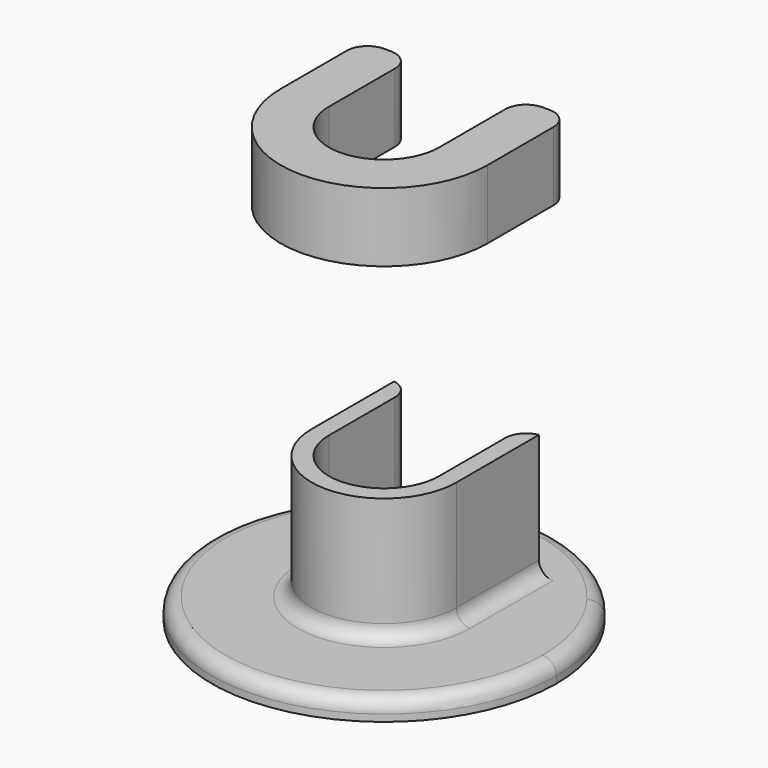
from build123d import *

# Parameters (mm, degrees)
F1_DEPTH = 3
F2_DEPTH = 18
F3_R     = 2
F4_R     = 3
F7_DEPTH = 10
F8_R     = 3


with BuildPart() as f1:
    # F0 (on Top) → F1 (new body)
    with BuildSketch(Plane.XY):
        with BuildLine():
            ThreePointArc((-20, 15), (-7.9056941504, -23.7170824513), (25, 0))
            ThreePointArc((25, 0), (23.7170824513, 7.9056941504), (20, 15))
            Line((20, 15), (10.5, 15))
            Line((10.5, 15), (10.5, 0))
            ThreePointArc((10.5, 0), (0, -10.5), (-10.5, 0))
            Line((-10.5, 0), (-10.5, 15))
            Line((-10.5, 15), (-20, 15))
        make_face()
        with BuildLine():
            Line((10.5, 15), (20, 15))
            ThreePointArc((20, 15), (0, 25), (-20, 15))
            Line((-20, 15), (-10.5, 15))
            Line((-10.5, 15), (-8, 15))
            Line((-8, 15), (8, 15))
            Line((8, 15), (10.5, 15))
        make_face()
        with BuildLine():
            ThreePointArc((-8, 0), (0, -8), (8, 0))
            ThreePointArc((8, 0), (0, 8), (-8, 0))
        make_face()
        with BuildLine():
            Line((8, 0), (8, 6.8007352544))
            ThreePointArc((8, 6.8007352544), (0, 10.5), (-8, 6.8007352544))
            Line((-8, 6.8007352544), (-8, 0))
            ThreePointArc((-8, 0), (0, 8), (8, 0))
        make_face()
        with BuildLine():
            ThreePointArc((-10.5, 0), (0, -10.5), (10.5, 0))
            ThreePointArc((10.5, 0), (9.8552016722, 3.6228441865), (8, 6.8007352544))
            Line((8, 6.8007352544), (8, 0))
            ThreePointArc((8, 0), (0, -8), (-8, 0))
            Line((-8, 0), (-8, 6.8007352544))
            ThreePointArc((-8, 6.8007352544), (-9.8552016722, 3.6228441865), (-10.5, 0))
        make_face()
        with BuildLine():
            Line((-8, 15), (-10.5, 15))
            Line((-10.5, 15), (-10.5, 0))
            ThreePointArc((-10.5, 0), (-9.8552016722, 3.6228441865), (-8, 6.8007352544))
            Line((-8, 6.8007352544), (-8, 15))
        make_face()
        with BuildLine():
            Line((8, 6.8007352544), (8, 15))
            Line((8, 15), (-8, 15))
            Line((-8, 15), (-8, 6.8007352544))
            ThreePointArc((-8, 6.8007352544), (0, 10.5), (8, 6.8007352544))
        make_face()
        with BuildLine():
            Line((10.5, 0), (10.5, 15))
            Line((10.5, 15), (8, 15))
            Line((8, 15), (8, 6.8007352544))
            ThreePointArc((8, 6.8007352544), (9.8552016722, 3.6228441865), (10.5, 0))
        make_face()
    extrude(amount=-F1_DEPTH)

    # F0 (on Top) → F2 (join)
    with BuildSketch(Plane.XY):
        with BuildLine():
            Line((10.5, 0), (10.5, 15))
            Line((10.5, 15), (8, 15))
            Line((8, 15), (8, 6.8007352544))
            ThreePointArc((8, 6.8007352544), (9.8552016722, 3.6228441865), (10.5, 0))
        make_face()
        with BuildLine():
            ThreePointArc((-10.5, 0), (0, -10.5), (10.5, 0))
            ThreePointArc((10.5, 0), (9.8552016722, 3.6228441865), (8, 6.8007352544))
            Line((8, 6.8007352544), (8, 0))
            ThreePointArc((8, 0), (0, -8), (-8, 0))
            Line((-8, 0), (-8, 6.8007352544))
            ThreePointArc((-8, 6.8007352544), (-9.8552016722, 3.6228441865), (-10.5, 0))
        make_face()
        with BuildLine():
            Line((-8, 15), (-10.5, 15))
            Line((-10.5, 15), (-10.5, 0))
            ThreePointArc((-10.5, 0), (-9.8552016722, 3.6228441865), (-8, 6.8007352544))
            Line((-8, 6.8007352544), (-8, 15))
        make_face()
    extrude(amount=F2_DEPTH)

    # F3
    f3_edges = [f1.edges().sort_by_distance(p)[0] for p in [
        (-25, 0, 0),
        (0, -10.5, 0),
        (10.5, 7.5, 0),
        (-10.5, 7.5, 0),
    ]]
    fillet(f3_edges, radius=F3_R)

    # F4
    f4_edges = [f1.edges().sort_by_distance(p)[0] for p in [
        (-8, 15, 9),
        (8, 15, 9),
    ]]
    fillet(f4_edges, radius=F4_R)


with BuildPart() as f7:
    # F6 (on offset) → F7 (new body)
    with BuildSketch(Plane.XY.offset(50)):
        with BuildLine():
            Line((-15, 15), (-15, 0))
            ThreePointArc((-15, 0), (-13.1339255366, 7.2456883731), (-8, 12.6885775404))
            Line((-8, 12.6885775404), (-8, 15))
            Line((-8, 15), (-15, 15))
        make_face()
        with BuildLine():
            ThreePointArc((-8, 12.6885775404), (-13.1339255366, 7.2456883731), (-15, 0))
            ThreePointArc((-15, 0), (0, -15), (15, 0))
            ThreePointArc((15, 0), (13.1339255366, 7.2456883731), (8, 12.6885775404))
            Line((8, 12.6885775404), (8, 0))
            ThreePointArc((8, 0), (0, -8), (-8, 0))
            Line((-8, 0), (-8, 12.6885775404))
        make_face()
        with BuildLine():
            ThreePointArc((8, 12.6885775404), (13.1339255366, 7.2456883731), (15, 0))
            Line((15, 0), (15, 15))
            Line((15, 15), (8, 15))
            Line((8, 15), (8, 12.6885775404))
        make_face()
    extrude(amount=F7_DEPTH)

    # F8
    f8_edges = [f7.edges().sort_by_distance(p)[0] for p in [
        (-8, 15, 55),
        (8, 15, 55),
        (-15, 15, 55),
        (15, 15, 55),
    ]]
    fillet(f8_edges, radius=F8_R)


solid = Compound([f1.part, f7.part])
